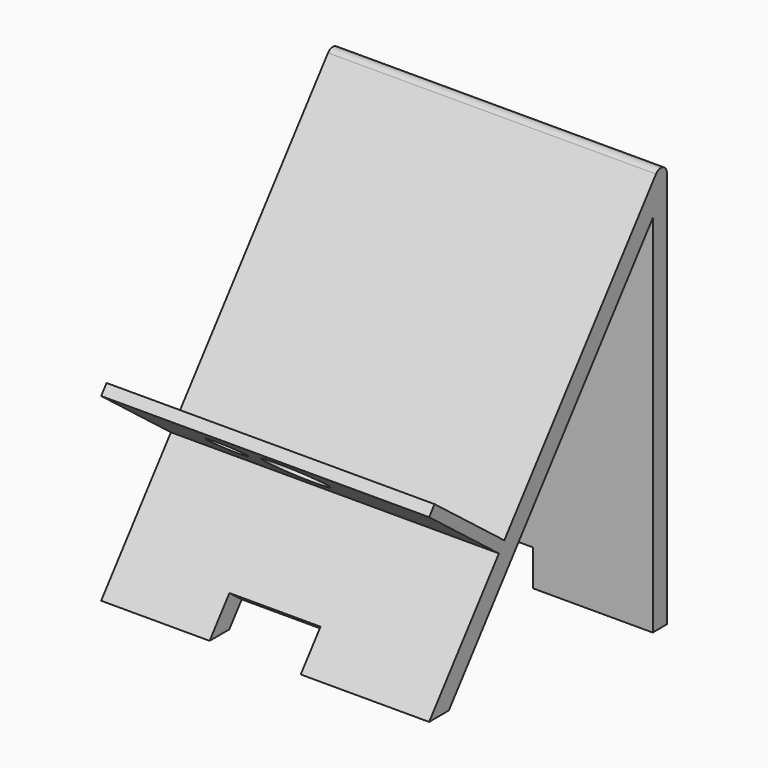
from build123d import *

# Parameters (mm, degrees)
F1_DEPTH      = 241.3
F1_DEPTH_BACK = 281.94
F2_R          = 46.8036250012
F2_R_2        = 29.082061138
F3_DEPTH      = 86.36
F4_W          = 145.3568041325
F4_H          = 64.5723461173
F5_DEPTH      = 78.74
F6_W          = 156.2250889838
F6_H          = 57.1747124195
F7_DEPTH      = 81.28
F8_W          = 156.9080613554
F8_H          = 28.0602325869
F9_DEPTH      = 40.64
F10_TEXT_SIZE = 183.4302908726
F11_DEPTH     = 7.62
F12_R         = 12.1177057122


# Not quite as in the source:
# - Text() gives the source's letters only with a copy of the font that has no kerning and outlines rounded to 1/6400 em; it was checked with that copy


with BuildPart() as f1:
    # F0 (on Right) → F1 (new body, two sides)
    with BuildSketch(Plane.YZ) as f1_sk:
        Polygon((181.7104965448, -420.9338724613), (181.7104965448, 192.7392631769), (-142.4618316498, -226.8837835111), (-153.2626566118, -240.864850626), (-292.3717796803, -420.9338724613), (-253.0980408192, -420.9338724613), (153.6525456952, 105.5821361871), (153.6525456952, -476.7968356609), (181.7104965448, -476.438999176), align=None)
        Polygon((-153.2626566118, -240.864850626), (-142.4618316498, -226.8837835111), (-281.5709547183, -119.4175023948), (-292.3717796803, -133.3985695098), align=None)
    extrude(amount=F1_DEPTH)
    extrude(f1_sk.sketch, amount=-F1_DEPTH_BACK)

    # F2 (on face) → F3 (cut)
    with BuildSketch(Plane(origin=(0, -173.8119297897, -224.9898747843), x_dir=(1, 0, 0), z_dir=(0, -0.6113508539, -0.7913596739))):
        with Locations((-26.0912720114, 63.2995516062)):
            Circle(F2_R)
        with Locations((-135.2015435696, 64.9607777596)):
            Circle(F2_R_2)
    extrude(amount=-F3_DEPTH, mode=Mode.SUBTRACT)

    # F4 (on face) → F5 (cut)
    with BuildSketch(Plane(origin=(0, 20.5492731779, -15.8749758417), x_dir=(1, 0, 0), z_dir=(0, -0.7913596739, 0.6113508539))):
        with Locations((-36.2294688821, -479.5656561386)):
            Rectangle(F4_W, F4_H)
    extrude(amount=-F5_DEPTH, mode=Mode.SUBTRACT)

    # F6 (on face) → F7 (cut)
    with BuildSketch(Plane(origin=(0, 181.7104965448, 0), x_dir=(-1, 0, 0), z_dir=(0, 1, 0))):
        with Locations((28.0032064766, -447.8516429663)):
            Rectangle(F6_W, F6_H)
    extrude(amount=-F7_DEPTH, mode=Mode.SUBTRACT)

    # F8 (on face) → F9 (cut)
    with BuildSketch(Plane(origin=(0, 6.104817215, -478.6785825069), x_dir=(1, 0, 0), z_dir=(0, 0.0127524419, -0.9999186843))):
        with Locations((-28.3446926624, -161.5898436951)):
            Rectangle(F8_W, F8_H)
    extrude(amount=-F9_DEPTH, mode=Mode.SUBTRACT)

    # F10 (on face) → F11 (join)
    with BuildSketch(Plane(origin=(0, 181.7104965448, 0), x_dir=(-1, 0, 0), z_dir=(0, 1, 0))):
        with Locations((-207.743787592, -106.2476515018)):
            Text('EAHS', F10_TEXT_SIZE, font='Open Sans', text_align=(TextAlign.LEFT, TextAlign.BOTTOM))
    extrude(amount=F11_DEPTH)

    # F12
    f12_edges = [f1.edges().sort_by_distance(p)[0] for p in [
        (-20.32, 181.710497, 192.739263),
    ]]
    fillet(f12_edges, radius=F12_R)


solid = f1.part
